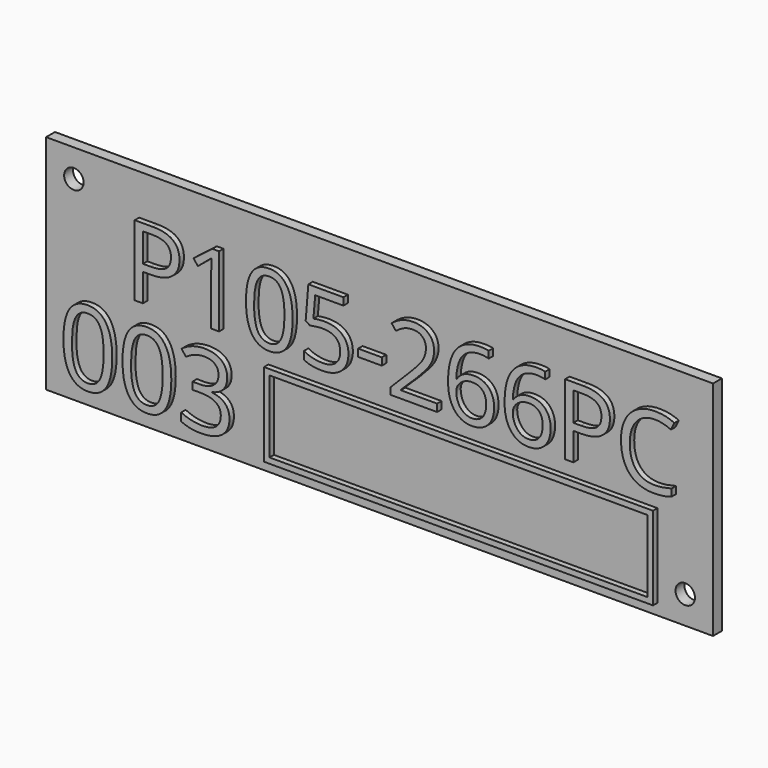
from build123d import *

# Parameters (mm, degrees)
F0_W         = 120
F0_H         = 40
F1_DEPTH     = 2
F3_D         = 3.5
F4_TEXT_SIZE = 17.7871654484
F5_DEPTH     = 1
F6_TEXT_SIZE = 18.5894526641
F7_DEPTH     = 1
F8_W         = 70
F8_H         = 15
F8_W_2       = 68
F8_H_2       = 13
F9_DEPTH     = 1


# Not quite as in the source:
# - Text() gives the source's letters only with a copy of the font that has no kerning and outlines rounded to 1/6400 em; it was checked with that copy


with BuildPart() as f1:
    # F0 (on Front) → F1 (new body)
    with BuildSketch(Plane.XZ):
        Rectangle(F0_W, F0_H)
    extrude(amount=F1_DEPTH)

    # F3 (through all)
    with Locations(Plane.XZ.offset(2)):
        with Locations((-55, 15), (55, -15)):
            Hole(F3_D / 2)

    # F4 (on face) → F5 (join)
    with BuildSketch(Plane.XZ.offset(2)):
        with Locations((-45, 0)):
            Text('P105-266PC', F4_TEXT_SIZE, font='Open Sans', text_align=(TextAlign.LEFT, TextAlign.BOTTOM))
    extrude(amount=F5_DEPTH)

    # F6 (on face) → F7 (join)
    with BuildSketch(Plane.XZ.offset(2)):
        with Locations((-57, -17)):
            Text('003', F6_TEXT_SIZE, font='Open Sans', text_align=(TextAlign.LEFT, TextAlign.BOTTOM))
    extrude(amount=F7_DEPTH)

    # F8 (on face) → F9 (join)
    with BuildSketch(Plane.XZ.offset(2)):
        with Locations((15, -10.5)):
            Rectangle(F8_W, F8_H)
        with Locations((15, -10.5)):
            Rectangle(F8_W_2, F8_H_2, mode=Mode.SUBTRACT)
    extrude(amount=F9_DEPTH)


solid = f1.part
